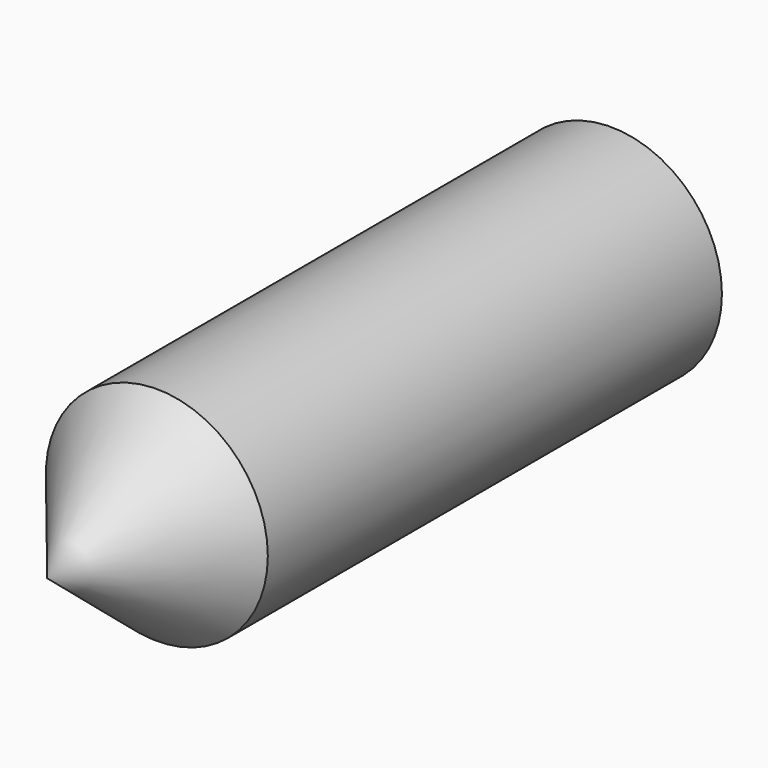
from build123d import *

# Parameters (mm, degrees)
F0_R     = 29.796459214
F0_R_2   = 12.7
F1_DEPTH = 152.4
F2_R     = 29.796459214


# Not quite as in the source:
# - an extrude whose draft closes it to a point is written as a loft to that point


with BuildPart() as f1:
    # F0 (on Front) → F1 (new body)
    with BuildSketch(Plane.XZ):
        Circle(F0_R)
        Circle(F0_R_2, mode=Mode.SUBTRACT)
    extrude(amount=F1_DEPTH)

    # F2 (on face) → F3 section 0
    with BuildSketch(Plane.XZ.offset(152.4), mode=Mode.PRIVATE) as f3_s0:
        Circle(F2_R)
    loft([f3_s0.sketch, Vertex(0, -189.1955627582, 0)], ruled=True)


solid = f1.part
